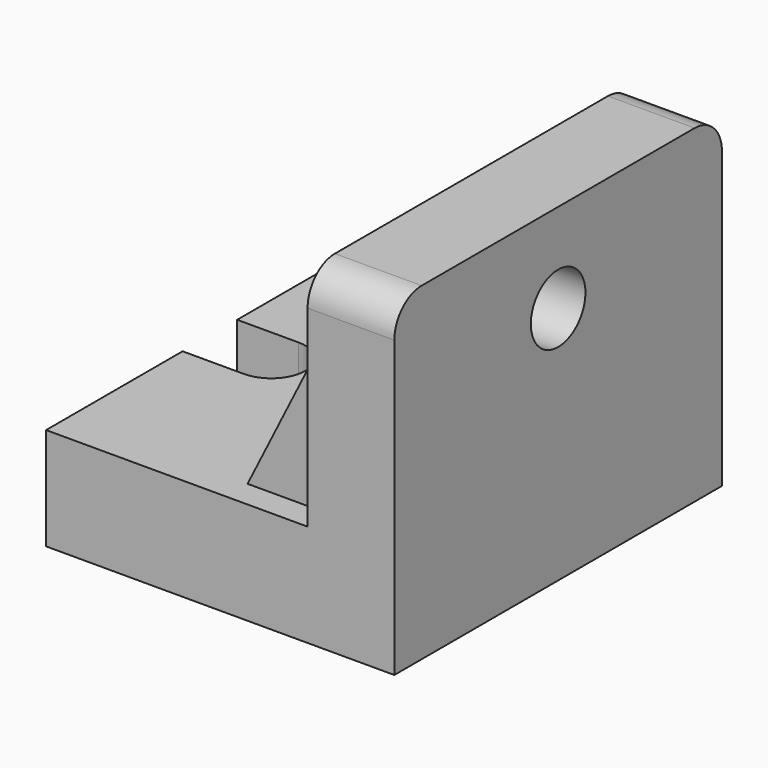
from build123d import *

# Parameters (mm, degrees)
F1_DEPTH = 30
F2_R     = 5
F3_DEPTH = 12.7077577636
F5_DEPTH = 15.0035852566
F8_DEPTH = 8
F11_R    = 5


# Not quite as in the source:
# - a pattern or mirror of a feature is missing from the dataset's text; its kind, count and spacing are read off the source's solid
# - the program builds the solid bodies; features that only make, move or delete a surface that nothing else refers to are left out


with BuildPart() as f1:
    # F0 (on Front) → F1 (new body, symmetric)
    with BuildSketch(Plane.XZ):
        Polygon((-51.0283857584, 15.0035852566), (-51.0283857584, 0), (0, 0), (0, 48.1919869781), (-12.7077577636, 48.1919869781), (-12.7077577636, 15.0035852566), align=None)
    extrude(amount=F1_DEPTH, both=True)

    # F2 (on face) → F3 (cut, through all)
    with BuildSketch(Plane.YZ):
        with Locations((0, 35.1077616215)):
            Circle(F2_R)
    extrude(amount=-F3_DEPTH, mode=Mode.SUBTRACT)

    # F4 (on face) → F5 (cut, through all)
    with BuildSketch(Plane.XY.offset(15.0035852566)):
        with BuildLine():
            ThreePointArc((-42.0283857584, -5), (-38.4928518525, -3.5355339059), (-37.0283857584, 0))
            ThreePointArc((-37.0283857584, 0), (-38.4928518525, 3.5355339059), (-42.0283857584, 5))
            ThreePointArc((-42.0283857584, 5), (-47.0283857584, 0), (-42.0283857584, -5))
        make_face()
        with BuildLine():
            ThreePointArc((-42.0283857584, -5), (-47.0283857584, 0), (-42.0283857584, 5))
            Line((-42.0283857584, 5), (-51.0283857584, 5))
            Line((-51.0283857584, 5), (-51.0283857584, -5))
            Line((-51.0283857584, -5), (-42.0283857584, -5))
        make_face()
    extrude(amount=-F5_DEPTH, mode=Mode.SUBTRACT)

    # F7 (on offset) → F8 (join)
    with BuildSketch(Plane.XZ.offset(18)):
        Polygon((-12.7077577636, 39.0035852566), (-24.7077577636, 15.0035852566), (-12.7077577636, 15.0035852566), align=None)
    f8 = extrude(amount=F8_DEPTH)

    # F8_copies: F8 across plane
    add(f8.mirror(Plane.ZX))

    # F11
    f11_edges = [f1.edges().sort_by_distance(p)[0] for p in [
        (-6.353879, 30, 48.191987),
        (-6.353879, -30, 48.191987),
    ]]
    fillet(f11_edges, radius=F11_R)


solid = f1.part
